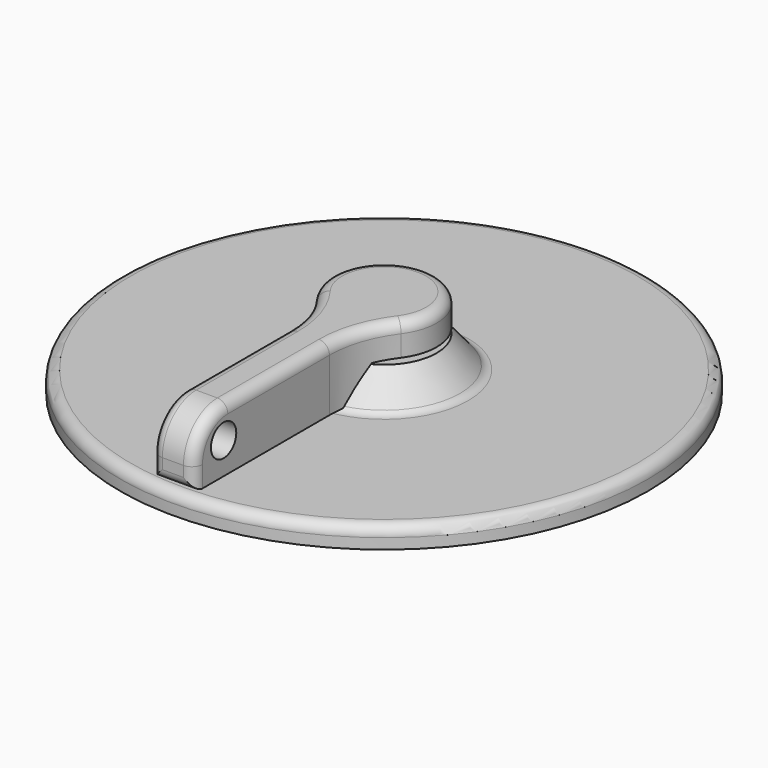
from build123d import *

# Parameters (mm, degrees)
F0_R      = 25
F1_DEPTH  = 2
F3_R      = 7.5
F4_DEPTH  = 3
F4_TAPER  = 40
F5_T      = 2
F2_R      = 3
F6_DEPTH  = 5.001
F8_R      = 2.5
F9_DEPTH  = 3
F10_R     = 3.1
F11_DEPTH = 1.5
F11_TAPER = 20
F13_R     = 4.9827011065
F14_DEPTH = 3
F15_DEPTH = 2
F16_R     = 10
F17_R     = 4
F18_R     = 1.5
F19_DEPTH = 27.001
F20_R     = 1
F21_R     = 1


# Not quite as in the source:
# - a shell that OpenCascade refuses in one call is made with other operations: the cavity is built on its own and cut out


with BuildPart() as f1:
    # F0 (on Top) → F1 (new body)
    with BuildSketch(Plane.XY):
        Circle(F0_R)
    extrude(amount=F1_DEPTH)

    # F3 (on face) → F4 (join)
    with BuildSketch(Plane.XY.offset(2)):
        Circle(F3_R)
    extrude(amount=F4_DEPTH, taper=F4_TAPER)

    # F5: shell of thickness 2, made by hand


with BuildPart() as f5_core1:
    # F5_t2: copy of F1
    add(f1.part)

    # the walls: a layer under each face that stays
    f5_faces = [f5_core1.faces().sort_by_distance(p)[0] for p in [
        (-25, 0, 1),
        (-16.6666666667, -16.6666666667, 2),
        (-6.2413505532, 0, 3.5),
        (0, 0, 5),
    ]]
    thicken(f5_faces, amount=-F5_T, mode=Mode.SUBTRACT)

    # F5_s3 → F5_t4 (revolve, cut)
    with BuildSketch(Plane.XZ):
        Polygon((7.5153208889, 2.0328557522), (7.5, 0), (6.5673846837, 0), (5.9679111138, 0.7144247806), align=None)
    revolve(axis=Axis((0, 0, 2), (0, 0, -1)), mode=Mode.SUBTRACT)


with BuildPart() as f1_1:
    add(f1.part)

    # what is left inside the walls is the cavity
    f5_cavity = [f5_core1.part.solids().sort_by_distance(p)[0] for p in [
        (0, -2.189128, 0.02),
    ]]
    add(f5_cavity, mode=Mode.SUBTRACT)

    # F2 (on Top) → F6 (cut, through all)
    with BuildSketch(Plane.XY):
        Circle(F2_R)
    extrude(amount=F6_DEPTH, mode=Mode.SUBTRACT)

    # F21
    f21_edges = [f1_1.edges().sort_by_distance(p)[0] for p in [
        (-25, 0, 2),
        (-7.5, 0, 2),
    ]]
    fillet(f21_edges, radius=F21_R)


with BuildPart() as f9:
    # F8 (on offset) → F9 (new body)
    with BuildSketch(Plane.XY.offset(5.5)):
        Circle(F8_R)
    extrude(amount=-F9_DEPTH)

    # F10 (on face) → F11 (join)
    with BuildSketch(Plane(origin=(0, 0, 2.5), x_dir=(1, 0, 0), z_dir=(0, 0, -1))):
        Circle(F10_R)
    extrude(amount=F11_DEPTH, taper=F11_TAPER)

    # F13 (on offset) → F14 (join)
    with BuildSketch(Plane.XY.offset(5.5)):
        Circle(F13_R)
    extrude(amount=F14_DEPTH)

    # F12 (on Right) → F15 (join, symmetric)
    with BuildSketch(Plane.YZ):
        Polygon((-4.9827011065, 5.5), (-2.5, 5.5), (0, 5.5), (0, 8.5), (-25, 8.5), (-25, 2.5), (-7.5, 2.5), align=None)
    extrude(amount=F15_DEPTH, both=True)

    # F16 (call 1 of 2: OpenCascade refuses the feature's edges together)
    f16_edges = [f9.edges().sort_by_distance(p)[0] for p in [
        (2, -4.563695, 7),
    ]]
    fillet(f16_edges, radius=F16_R)

    # F16#2 (call 2 of 2)
    f16_2_edges = [f9.edges().sort_by_distance(p)[0] for p in [
        (-2, -4.563695, 7),
    ]]
    fillet(f16_2_edges, radius=F16_R)

    # F17
    f17_edges = [f9.edges().sort_by_distance(p)[0] for p in [
        (0, -25, 8.5),
    ]]
    fillet(f17_edges, radius=F17_R)

    # F18 (on face) → F19 (cut, through all)
    with BuildSketch(Plane.YZ.offset(2)):
        with Locations((-21.5, 5.5)):
            Circle(F18_R)
    extrude(amount=-F19_DEPTH, mode=Mode.SUBTRACT)

    # F20
    f20_edges = [f9.edges().sort_by_distance(p)[0] for p in [
        (-2, -14.985569, 8.5),
        (0, -21, 8.5),
        (-2.510733, -5.816172, 8.5),
        (2, -14.985569, 8.5),
        (0, 4.982701, 8.5),
        (2.510733, -5.816172, 8.5),
        (-2, -23.828427, 7.328427),
        (0, -25, 4.5),
        (2, -23.828427, 7.328427),
        (-2, -25, 3.5),
        (0, -25, 2.5),
        (2, -25, 3.5),
    ]]
    fillet(f20_edges, radius=F20_R)


solid = Compound([f1_1.part, f9.part])
